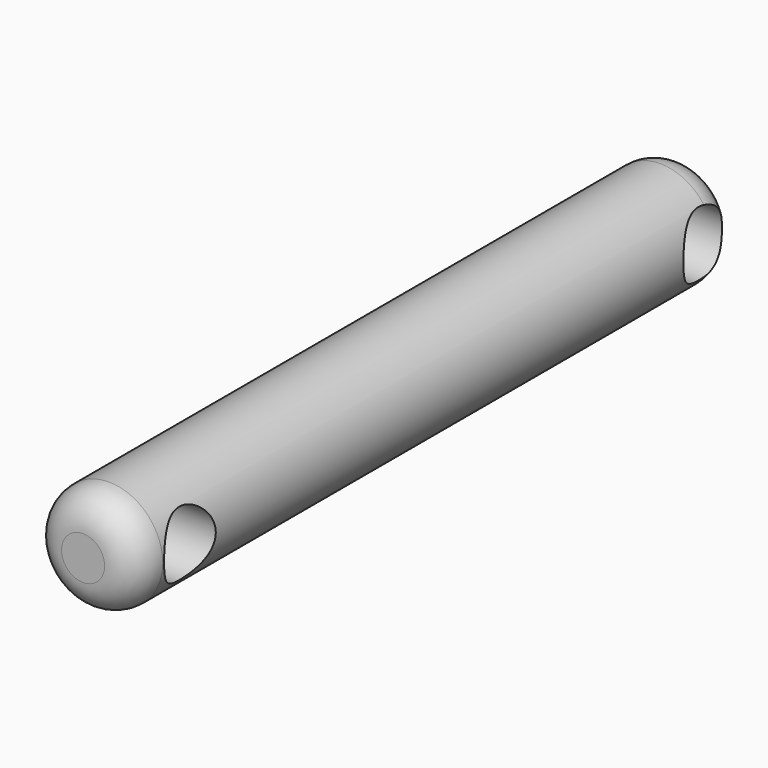
from build123d import *

# Parameters (mm, degrees)
F0_R     = 10
F1_DEPTH = 140
F2_R     = 6
F3_DEPTH = 200
F5_R     = 6
F6_DEPTH = 12.5
F7_R     = 6


# Not quite as in the source:
# - a fillet or chamfer that OpenCascade refuses, or shapes differently, is made with other operations: its cross-section is extruded or revolved along the edge and cut away or added


with BuildPart() as f1:
    # F0 (on Front) → F1 (new body)
    with BuildSketch(Plane.XZ):
        Circle(F0_R)
    extrude(amount=F1_DEPTH)

    # F2 (on Right) → F3 (cut, symmetric)
    with BuildSketch(Plane.YZ):
        with Locations((-7.1659120997, 0)):
            Circle(F2_R)
    extrude(amount=F3_DEPTH, both=True, mode=Mode.SUBTRACT)

    # F4: fillet of radius 6 on 1 edges, made by hand

    # F4_s1 → F4_t2 (revolve, cut)
    with BuildSketch(Plane.XY):
        with BuildLine():
            ThreePointArc((10, -6), (8.2426406871, -1.7573593129), (4, 0))
            Line((4, 0), (10, 0))
            Line((10, 0), (10, -6))
        make_face()
    revolve(axis=Axis((0, 0, 0), (0, -1, 0)), mode=Mode.SUBTRACT)

    # F5 (on Right) → F6 (cut, symmetric)
    with BuildSketch(Plane.YZ):
        with Locations((-127.698, 0)):
            Circle(F5_R)
    extrude(amount=F6_DEPTH, both=True, mode=Mode.SUBTRACT)

    # F7
    f7_edges = [f1.edges().sort_by_distance(p)[0] for p in [
        (-10, -140, 0),
    ]]
    fillet(f7_edges, radius=F7_R)


solid = f1.part
